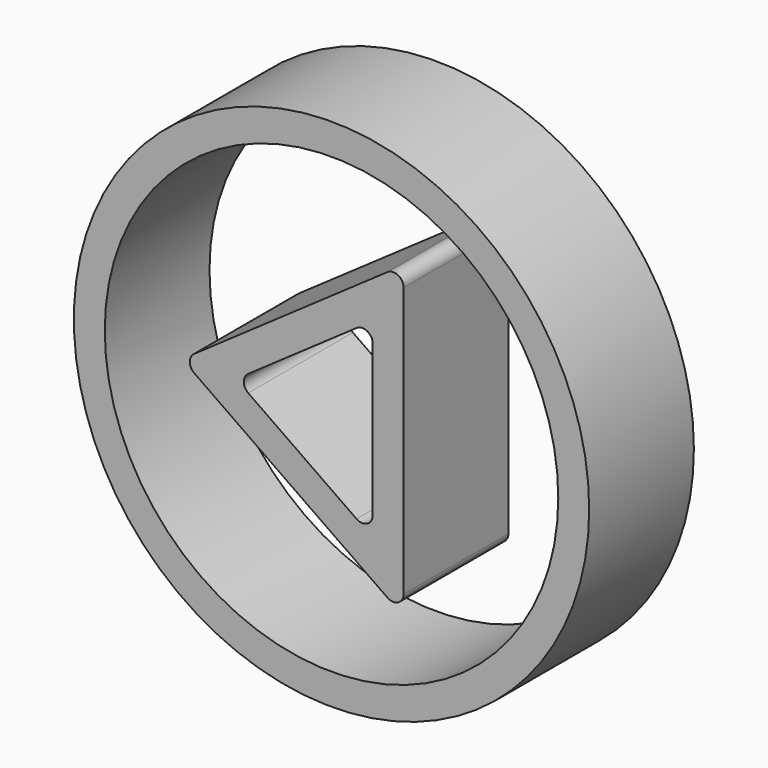
from build123d import *

# Parameters (mm, degrees)
F0_R     = 50
F0_R_2   = 44
F1_DEPTH = 25.4
F2_DEPTH = 25.4
F5_DEPTH = 25.4
F6_R     = 2


# Not quite as in the source:
# - a feature names something its author has since deleted; it is built from what else it names


with BuildPart() as f1:
    # F0 (on Front) → F1 (new body)
    with BuildSketch(Plane.XZ):
        Circle(F0_R)
        Circle(F0_R_2, mode=Mode.SUBTRACT)
    extrude(amount=F1_DEPTH)


with BuildPart() as f2:
    # F0 (on Front) → F2 (new body)
    with BuildSketch(Plane.XZ):
        Polygon((-29, 0), (0, 0), (14, 0), (14, 30), align=None)
    extrude(amount=F2_DEPTH)

    # F3: F2 across face


with BuildPart() as f2_1:
    add(f2.part)
    add(f2.part.mirror(Plane(origin=(-7.5, -12.7, 0), x_dir=(1, 0, 0), z_dir=(0, 0, -1))))

    # F4 (on face) → F5 (cut)
    with BuildSketch(Plane.XZ.offset(25.4)):
        Polygon((8, -18.4980129885), (8, 18.4980129885), (-18.5138186169, 0), align=None)
    extrude(amount=-F5_DEPTH, mode=Mode.SUBTRACT)

    # F6
    f6_edges = [f2_1.edges().sort_by_distance(p)[0] for p in [
        (14, -12.7, -30),
        (-29, -12.7, 0),
        (14, -12.7, 30),
        (8, -12.7, 18.498013),
        (-18.513819, -12.7, 0),
        (8, -12.7, -18.498013),
    ]]
    fillet(f6_edges, radius=F6_R)


solid = Compound([f1.part, f2_1.part])
